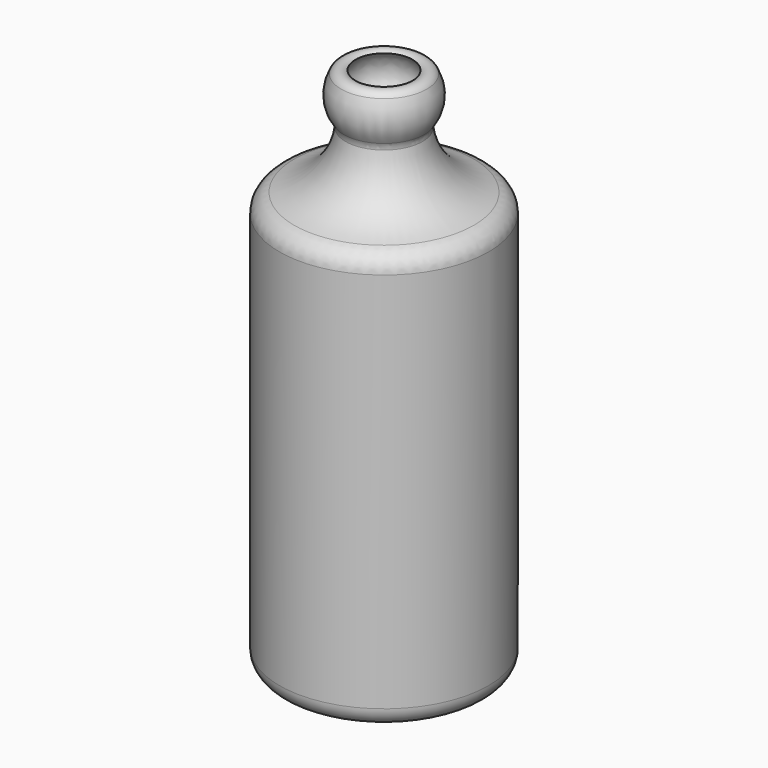
from build123d import *

# Parameters (mm, degrees)
F2_R = 6.35
F3_R = 6.35
F5_R = 3.175
F6_R = 6.35
F7_R = 6.35


# Not quite as in the source:
# - a fillet or chamfer that OpenCascade refuses, or shapes differently, is made with other operations: its cross-section is extruded or revolved along the edge and cut away or added


with BuildPart() as f1:
    # F0 (on Front) → F1 (revolve)
    with BuildSketch(Plane.XZ):
        with BuildLine():
            Line((31.75, 0), (0, 0))
            Line((0, 0), (0, -3.175))
            Line((0, -3.175), (34.925, -3.175))
            Line((34.925, -3.175), (34.925, 136.3257812379))
            ThreePointArc((34.925, 136.3257812379), (19.661541674, 142.3959842744), (12.7357473371, 157.2907450236))
            ThreePointArc((12.7357473371, 157.2907450236), (15.7038360971, 167.7283408709), (9.525, 176.6488196945))
            Line((9.525, 176.6488196945), (9.525, 172.749812895))
            ThreePointArc((9.525, 172.749812895), (12.7, 165.6502970665), (9.525, 158.5507812379))
            ThreePointArc((9.525, 158.5507812379), (15.875, 141.7502604126), (31.75, 133.35))
            Line((31.75, 133.35), (31.75, 0))
        make_face()
    revolve(axis=Axis((0, 0, 88.3244098473), (0, 0, -1)))

    # F2
    f2_edges = [f1.edges().sort_by_distance(p)[0] for p in [
        (-34.925, 0, 136.325781),
    ]]
    fillet(f2_edges, radius=F2_R)

    # F3
    f3_edges = [f1.edges().sort_by_distance(p)[0] for p in [
        (-34.925, 0, -3.175),
    ]]
    fillet(f3_edges, radius=F3_R)

    # F4: fillet of radius 3.175 on 1 edges, made by hand

    # F4_s1 → F4_t2 (revolve, cut)
    with BuildSketch(Plane.XZ):
        with BuildLine():
            ThreePointArc((14.2825038565, 171.8076794711), (12.1223989967, 173.382851233), (9.525, 172.749812895))
            Line((9.525, 172.749812895), (9.525, 176.6488196945))
            ThreePointArc((9.525, 176.6488196945), (12.2331604032, 174.5519671406), (14.2825038565, 171.8076794711))
        make_face()
    revolve(axis=Axis((0, 0, 176.6488196945), (0, 0, -1)), mode=Mode.SUBTRACT)

    # F5
    f5_edges = [f1.edges().sort_by_distance(p)[0] for p in [
        (-12.735747, 0, 157.290745),
    ]]
    fillet(f5_edges, radius=F5_R)

    # F6
    f6_edges = [f1.edges().sort_by_distance(p)[0] for p in [
        (-31.75, 0, 0),
    ]]
    fillet(f6_edges, radius=F6_R)

    # F7
    f7_edges = [f1.edges().sort_by_distance(p)[0] for p in [
        (-31.75, 0, 133.35),
    ]]
    fillet(f7_edges, radius=F7_R)


solid = f1.part
